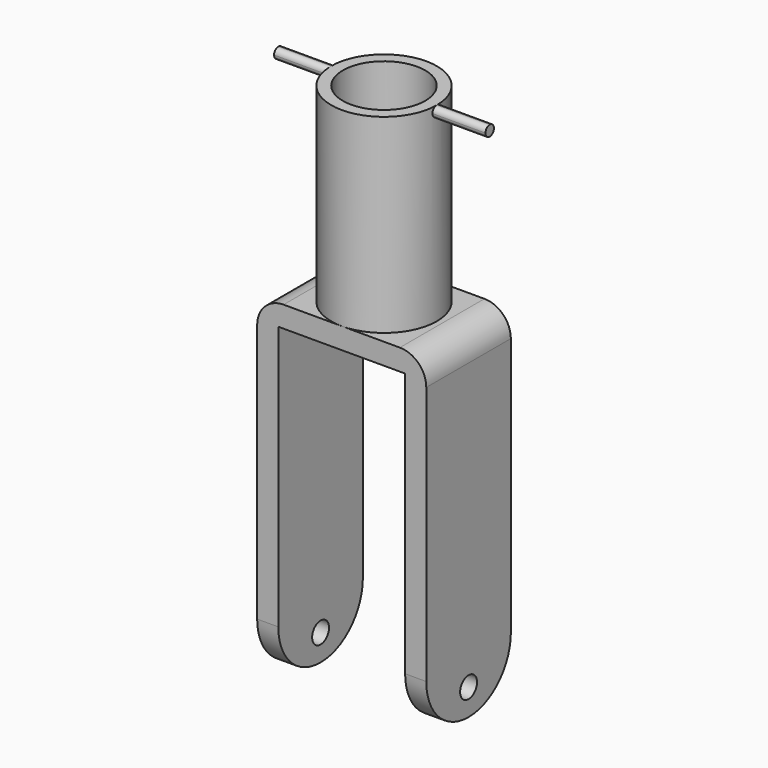
from build123d import *

# Parameters (mm, degrees)
F0_R      = 6.35
F0_R_2    = 0.635
F1_DEPTH  = 63.5
F3_DEPTH  = 1.27
F4_R      = 0.6349
F5_R      = 0.635
F6_DEPTH  = 40.64
F7_R      = 1.27
F8_DEPTH  = 25.4
F9_W      = 15.24
F9_H      = 38.1
F10_DEPTH = 12.7
F11_R     = 4.953
F11_R_2   = 0.635
F12_DEPTH = 25.4
F13_R     = 6.34999
F14_R     = 3.175


# Not quite as in the source:
# - a fillet or chamfer is up to 0.001 mm smaller than in the source, because OpenCascade refuses the exact size


with BuildPart() as f1:
    # F0 (on Top) → F1 (new body)
    with BuildSketch(Plane.XY):
        Circle(F0_R)
        Circle(F0_R_2, mode=Mode.SUBTRACT)
    extrude(amount=F1_DEPTH)

    # F2 (on face) → F3 (join)
    with BuildSketch(Plane.XY.offset(63.5)):
        with BuildLine():
            Line((6.3181702256, -0.635), (12.7, -0.635))
            Line((12.7, -0.635), (12.7, 0.635))
            Line((12.7, 0.635), (6.3181702256, 0.635))
            ThreePointArc((6.3181702256, 0.635), (6.3420375643, 0.3178986216), (6.35, 0))
            ThreePointArc((6.35, 0), (6.3420375643, -0.3178986216), (6.3181702256, -0.635))
        make_face()
        with BuildLine():
            Line((-12.7, -0.635), (-6.3181702256, -0.635))
            ThreePointArc((-6.3181702256, -0.635), (-6.35, 0), (-6.3181702256, 0.635))
            Line((-6.3181702256, 0.635), (-12.7, 0.635))
            Line((-12.7, 0.635), (-12.7, -0.635))
        make_face()
    extrude(amount=-F3_DEPTH)

    # F4 (radius 0.635 in the source; OpenCascade refuses exactly that, so slightly less here)
    f4_edges = [f1.edges().sort_by_distance(p)[0] for p in [
        (9.509085, 0.635, 63.5),
        (9.509085, -0.635, 63.5),
        (-9.509085, 0.635, 63.5),
        (-9.509085, -0.635, 63.5),
        (9.509085, 0.635, 62.23),
        (9.509085, -0.635, 62.23),
        (-9.509085, -0.635, 62.23),
        (-9.509085, 0.635, 62.23),
    ]]
    fillet(f4_edges, radius=F4_R)

    # F5 (on face) → F6 (join)
    with BuildSketch(Plane(origin=(0, 0, 0), x_dir=(1, 0, 0), z_dir=(0, 0, -1))):
        with BuildLine():
            ThreePointArc((0, -6.35), (-6.35, 0), (0, 6.35))
            Line((0, 6.35), (-10.16, 6.35))
            Line((-10.16, 6.35), (-10.16, -6.35))
            Line((-10.16, -6.35), (0, -6.35))
        make_face()
        with BuildLine():
            Line((10.16, -6.35), (10.16, 6.35))
            Line((10.16, 6.35), (0, 6.35))
            ThreePointArc((0, 6.35), (4.4901280605, 4.4901280605), (6.35, 0))
            ThreePointArc((6.35, 0), (4.4901280605, -4.4901280605), (0, -6.35))
            Line((0, -6.35), (10.16, -6.35))
        make_face()
        Circle(F5_R)
    extrude(amount=-F6_DEPTH)

    # F7 (on face) → F8 (cut)
    with BuildSketch(Plane(origin=(-10.16, 0, 0), x_dir=(0, -1, 0), z_dir=(-1, 0, 0))):
        with Locations((0, 3.175)):
            Circle(F7_R)
    extrude(amount=-F8_DEPTH, mode=Mode.SUBTRACT)

    # F9 (on face) → F10 (cut)
    with BuildSketch(Plane.XZ.offset(6.35)):
        with Locations((0, 19.05)):
            Rectangle(F9_W, F9_H)
    extrude(amount=-F10_DEPTH, mode=Mode.SUBTRACT)

    # F11 (on face) → F12 (cut, through all)
    with BuildSketch(Plane.XY.offset(63.5)):
        Circle(F11_R)
        Circle(F11_R_2, mode=Mode.SUBTRACT)
        Circle(F11_R_2)
    extrude(amount=-F12_DEPTH, mode=Mode.SUBTRACT)

    # F13 (radius 6.35 in the source; OpenCascade refuses exactly that, so slightly less here)
    f13_edges = [f1.edges().sort_by_distance(p)[0] for p in [
        (8.89, 6.35, 0),
        (8.89, -6.35, 0),
        (-8.89, -6.35, 0),
        (-8.89, 6.35, 0),
    ]]
    fillet(f13_edges, radius=F13_R)

    # F14
    f14_edges = [f1.edges().sort_by_distance(p)[0] for p in [
        (10.16, 0, 40.64),
        (-10.16, 0, 40.64),
    ]]
    fillet(f14_edges, radius=F14_R)


solid = f1.part
